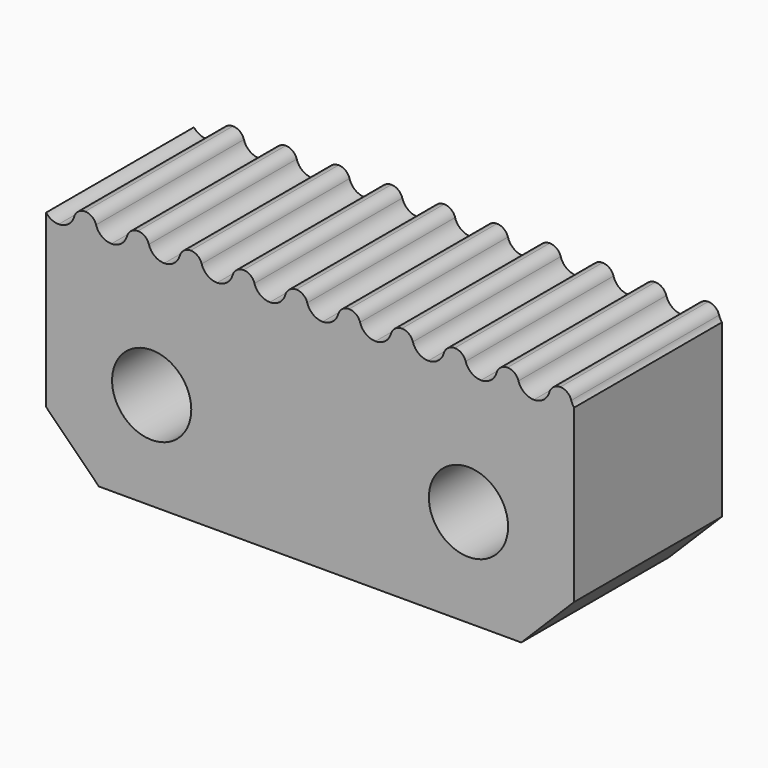
from build123d import *

# Parameters (mm, degrees)
F0_W         = 20
F0_H         = 9
F0_R         = 1.5
F1_DEPTH     = 7
F3_DEPTH     = 25
F4_SIZE      = 2
F5_TEXT_SIZE = 2.6725839331
F6_DEPTH     = 0.5


# Not quite as in the source:
# - Text() gives the source's letters only with a copy of the font that has no kerning and outlines rounded to 1/6400 em; it was checked with that copy


with BuildPart() as f1:
    # F0 (on Front) → F1 (new body)
    with BuildSketch(Plane.XZ):
        with Locations((12, 5.5)):
            Rectangle(F0_W, F0_H)
        with Locations((6, 4.7)):
            Circle(F0_R, mode=Mode.SUBTRACT)
        with Locations((18, 4.7)):
            Circle(F0_R, mode=Mode.SUBTRACT)
    extrude(amount=F1_DEPTH)

    # F2 (on face) → F3 (cut)
    with BuildSketch(Plane.XZ.offset(7)):
        with BuildLine():
            Line((4.4788280895, 10.63), (0, 10.63))
            Line((0, 10.63), (-1.6596260248, 10.63))
            Line((-1.6596260248, 10.63), (-1.5211719105, 9.25))
            ThreePointArc((-1.5211719105, 9.25), (-1.1557219003, 9.3718166701), (-0.9364518942, 9.6885400122))
            ThreePointArc((-0.9364518942, 9.6885400122), (-0.5211719105, 10), (-0.1058919268, 9.6885400122))
            ThreePointArc((-0.1058919268, 9.6885400122), (0.1133780793, 9.3718166701), (0.4788280895, 9.25))
            ThreePointArc((0.4788280895, 9.25), (0.8442780997, 9.3718166701), (1.0635481058, 9.6885400122))
            ThreePointArc((1.0635481058, 9.6885400122), (1.4788280895, 10), (1.8941080732, 9.6885400122))
            ThreePointArc((1.8941080732, 9.6885400122), (1.9371807124, 9.5805144244), (2, 9.4826445262))
            Line((2, 9.4826445262), (2, 10))
            Line((2, 10), (3.4788280895, 10))
            Line((3.4788280895, 10), (5.478828093, 10))
            Line((5.478828093, 10), (7.4788280895, 10))
            Line((7.4788280895, 10), (9.4788280895, 10))
            Line((9.4788280895, 10), (11.4788280895, 10))
            Line((11.4788280895, 10), (13.4788280895, 10))
            Line((13.4788280895, 10), (15.4788280895, 10))
            Line((15.4788280895, 10), (17.4788280895, 10))
            Line((17.4788280895, 10), (19.4788280895, 10))
            Line((19.4788280895, 10), (21.4788280895, 10))
            Line((21.4788280895, 10), (22, 10))
            Line((22, 10), (22, 9.4826445262))
            ThreePointArc((22, 9.4826445262), (22.2126515434, 9.3112397833), (22.4788280895, 9.25))
            ThreePointArc((22.4788280895, 9.25), (22.8442780997, 9.3718166701), (23.0635481058, 9.6885400122))
            ThreePointArc((23.0635481058, 9.6885400122), (23.4788280895, 10), (23.8941080732, 9.6885400122))
            ThreePointArc((23.8941080732, 9.6885400122), (24.1133780793, 9.3718166701), (24.4788280895, 9.25))
            Line((24.4788280895, 9.25), (24.4085397571, 10.63))
            Line((24.4085397571, 10.63), (22.9372018725, 10.63))
            Line((22.9372018725, 10.63), (4.4788280895, 10.63))
        make_face()
        with BuildLine():
            Line((2, 10), (2, 9.4826445262))
            ThreePointArc((2, 9.4826445262), (2.2126515434, 9.3112397833), (2.4788280895, 9.25))
            ThreePointArc((2.4788280895, 9.25), (2.8442780997, 9.3718166701), (3.0635481058, 9.6885400122))
            ThreePointArc((3.0635481058, 9.6885400122), (3.2192780997, 9.9134833367), (3.4788280895, 10))
            Line((3.4788280895, 10), (2, 10))
        make_face()
        with BuildLine():
            Line((5.478828093, 10), (3.4788280895, 10))
            ThreePointArc((3.4788280895, 10), (3.7383780793, 9.9134833367), (3.8941080732, 9.6885400122))
            ThreePointArc((3.8941080732, 9.6885400122), (4.1133780793, 9.3718166701), (4.4788280895, 9.25))
            ThreePointArc((4.4788280895, 9.25), (4.8442780997, 9.3718166701), (5.0635481058, 9.6885400122))
            ThreePointArc((5.0635481058, 9.6885400122), (5.2192781011, 9.9134833378), (5.478828093, 10))
        make_face()
        with BuildLine():
            Line((7.4788280895, 10), (5.478828093, 10))
            ThreePointArc((5.478828093, 10), (5.7383780807, 9.9134833357), (5.8941080732, 9.6885400122))
            ThreePointArc((5.8941080732, 9.6885400122), (6.1133780793, 9.3718166701), (6.4788280895, 9.25))
            ThreePointArc((6.4788280895, 9.25), (6.8442780997, 9.3718166701), (7.0635481058, 9.6885400122))
            ThreePointArc((7.0635481058, 9.6885400122), (7.2192780997, 9.9134833367), (7.4788280895, 10))
        make_face()
        with BuildLine():
            Line((9.4788280895, 10), (7.4788280895, 10))
            ThreePointArc((7.4788280895, 10), (7.7383780793, 9.9134833367), (7.8941080732, 9.6885400122))
            ThreePointArc((7.8941080732, 9.6885400122), (8.1133780793, 9.3718166701), (8.4788280895, 9.25))
            ThreePointArc((8.4788280895, 9.25), (8.8442780997, 9.3718166701), (9.0635481058, 9.6885400122))
            ThreePointArc((9.0635481058, 9.6885400122), (9.2192780997, 9.9134833367), (9.4788280895, 10))
        make_face()
        with BuildLine():
            Line((11.4788280895, 10), (9.4788280895, 10))
            ThreePointArc((9.4788280895, 10), (9.7383780793, 9.9134833367), (9.8941080732, 9.6885400122))
            ThreePointArc((9.8941080732, 9.6885400122), (10.1133780793, 9.3718166701), (10.4788280895, 9.25))
            ThreePointArc((10.4788280895, 9.25), (10.8442780997, 9.3718166701), (11.0635481058, 9.6885400122))
            ThreePointArc((11.0635481058, 9.6885400122), (11.2192780997, 9.9134833367), (11.4788280895, 10))
        make_face()
        with BuildLine():
            ThreePointArc((13.0635481058, 9.6885400122), (13.2192780997, 9.9134833367), (13.4788280895, 10))
            Line((13.4788280895, 10), (11.4788280895, 10))
            ThreePointArc((11.4788280895, 10), (11.7383780793, 9.9134833367), (11.8941080732, 9.6885400122))
            ThreePointArc((11.8941080732, 9.6885400122), (12.1133780793, 9.3718166701), (12.4788280895, 9.25))
            ThreePointArc((12.4788280895, 9.25), (12.8442780997, 9.3718166701), (13.0635481058, 9.6885400122))
        make_face()
        with BuildLine():
            ThreePointArc((15.0635481058, 9.6885400122), (15.2192780997, 9.9134833367), (15.4788280895, 10))
            Line((15.4788280895, 10), (13.4788280895, 10))
            ThreePointArc((13.4788280895, 10), (13.7383780793, 9.9134833367), (13.8941080732, 9.6885400122))
            ThreePointArc((13.8941080732, 9.6885400122), (14.1133780793, 9.3718166701), (14.4788280895, 9.25))
            ThreePointArc((14.4788280895, 9.25), (14.8442780997, 9.3718166701), (15.0635481058, 9.6885400122))
        make_face()
        with BuildLine():
            ThreePointArc((17.0635481058, 9.6885400122), (17.2192780997, 9.9134833367), (17.4788280895, 10))
            Line((17.4788280895, 10), (15.4788280895, 10))
            ThreePointArc((15.4788280895, 10), (15.7383780793, 9.9134833367), (15.8941080732, 9.6885400122))
            ThreePointArc((15.8941080732, 9.6885400122), (16.1133780793, 9.3718166701), (16.4788280895, 9.25))
            ThreePointArc((16.4788280895, 9.25), (16.8442780997, 9.3718166701), (17.0635481058, 9.6885400122))
        make_face()
        with BuildLine():
            ThreePointArc((19.0635481058, 9.6885400122), (19.2192780997, 9.9134833367), (19.4788280895, 10))
            Line((19.4788280895, 10), (17.4788280895, 10))
            ThreePointArc((17.4788280895, 10), (17.7383780793, 9.9134833367), (17.8941080732, 9.6885400122))
            ThreePointArc((17.8941080732, 9.6885400122), (18.1133780793, 9.3718166701), (18.4788280895, 9.25))
            ThreePointArc((18.4788280895, 9.25), (18.8442780997, 9.3718166701), (19.0635481058, 9.6885400122))
        make_face()
        with BuildLine():
            ThreePointArc((21.0635481058, 9.6885400122), (21.2192780997, 9.9134833367), (21.4788280895, 10))
            Line((21.4788280895, 10), (19.4788280895, 10))
            ThreePointArc((19.4788280895, 10), (19.7383780793, 9.9134833367), (19.8941080732, 9.6885400122))
            ThreePointArc((19.8941080732, 9.6885400122), (20.1133780793, 9.3718166701), (20.4788280895, 9.25))
            ThreePointArc((20.4788280895, 9.25), (20.8442780997, 9.3718166701), (21.0635481058, 9.6885400122))
        make_face()
        with BuildLine():
            ThreePointArc((21.8941080732, 9.6885400122), (21.9371807124, 9.5805144244), (22, 9.4826445262))
            Line((22, 9.4826445262), (22, 10))
            Line((22, 10), (21.4788280895, 10))
            ThreePointArc((21.4788280895, 10), (21.7383780793, 9.9134833367), (21.8941080732, 9.6885400122))
        make_face()
    extrude(amount=-F3_DEPTH, mode=Mode.SUBTRACT)

    # F4
    f4_edges = [f1.edges().sort_by_distance(p)[0] for p in [
        (2, -3.5, 1),
        (22, -3.5, 1),
    ]]
    chamfer(f4_edges, length=F4_SIZE)

    # F5 (on face) → F6 (cut)
    with BuildSketch(Plane(origin=(0, 0, 1), x_dir=(1, 0, 0), z_dir=(0, 0, -1))):
        with Locations((4.6930471435, 2.3462886456)):
            Text('ULTI*AKER', F5_TEXT_SIZE, font='Open Sans', font_style=FontStyle.BOLD, text_align=(TextAlign.LEFT, TextAlign.BOTTOM))
    extrude(amount=-F6_DEPTH, mode=Mode.SUBTRACT)


solid = f1.part
